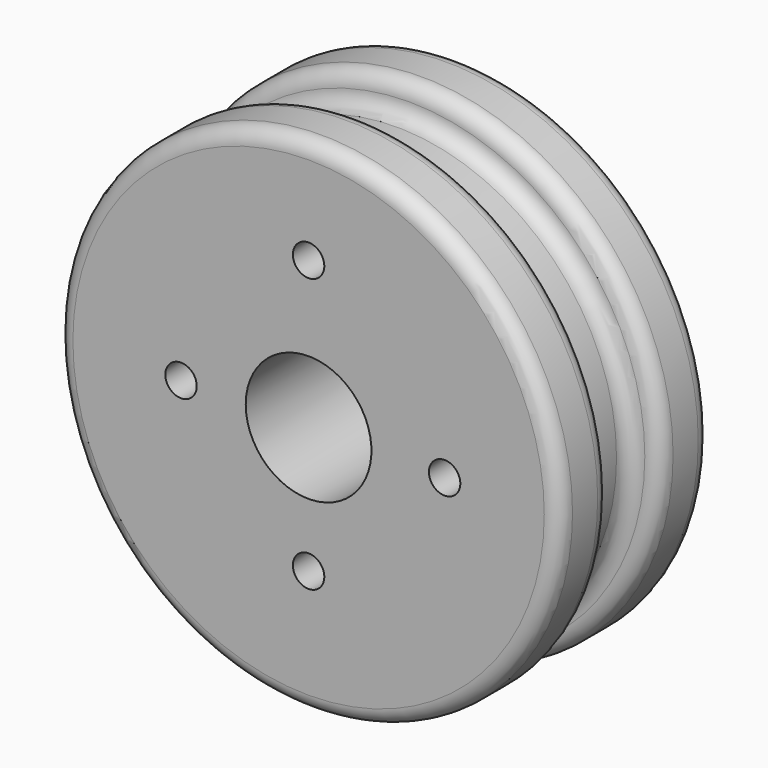
from build123d import *

# Parameters (mm, degrees)
F0_R     = 25.4
F1_DEPTH = 6.35
F2_R     = 22.225
F3_DEPTH = 12.7
F4_R     = 25.4
F4_R_2   = 22.225
F5_DEPTH = 6.35
F7_D     = 3.175
F7_DEPTH = 3.175
F7_TIP   = 0.9538662327
F8_D     = 12.7
F9_R     = 1.58749


# Not quite as in the source:
# - a fillet or chamfer is up to 0.001 mm smaller than in the source, because OpenCascade refuses the exact size


with BuildPart() as f1:
    # F0 (on Front) → F1 (new body)
    with BuildSketch(Plane.XZ):
        Circle(F0_R)
    extrude(amount=F1_DEPTH)

    # F2 (on Front) → F3 (join)
    with BuildSketch(Plane.XZ):
        Circle(F2_R)
    extrude(amount=F3_DEPTH)

    # F4 (on face) → F5 (join)
    with BuildSketch(Plane.XZ.offset(12.7)):
        Circle(F4_R)
        Circle(F4_R_2, mode=Mode.SUBTRACT)
        Circle(F4_R_2)
    extrude(amount=F5_DEPTH)

    # F7
    with Locations(Plane.XZ.offset(19.05)):
        with Locations((0, 14.8734748363), (13.7439081445, 0), (0, -12.7705568448), (-12.8878084943, 0)):
            Hole(F7_D / 2, depth=F7_DEPTH)
            with Locations((0, 0, -(F7_DEPTH + F7_TIP / 2))):  # 118° drill point
                Cone(0, F7_D / 2, F7_TIP, mode=Mode.SUBTRACT)

    # F8 (through all)
    with Locations(Plane.XZ.offset(19.05)):
        with Locations((0, 0)):
            Hole(F8_D / 2)

    # F9 (radius 1.5875 in the source; OpenCascade refuses exactly that, so slightly less here)
    f9_edges = [f1.edges().sort_by_distance(p)[0] for p in [
        (-25.4, 0, 0),
        (-25.4, -6.35, 0),
        (-22.225, -6.35, 0),
        (-22.225, -12.7, 0),
        (-25.4, -12.7, 0),
        (-25.4, -19.05, 0),
    ]]
    fillet(f9_edges, radius=F9_R)


solid = f1.part
